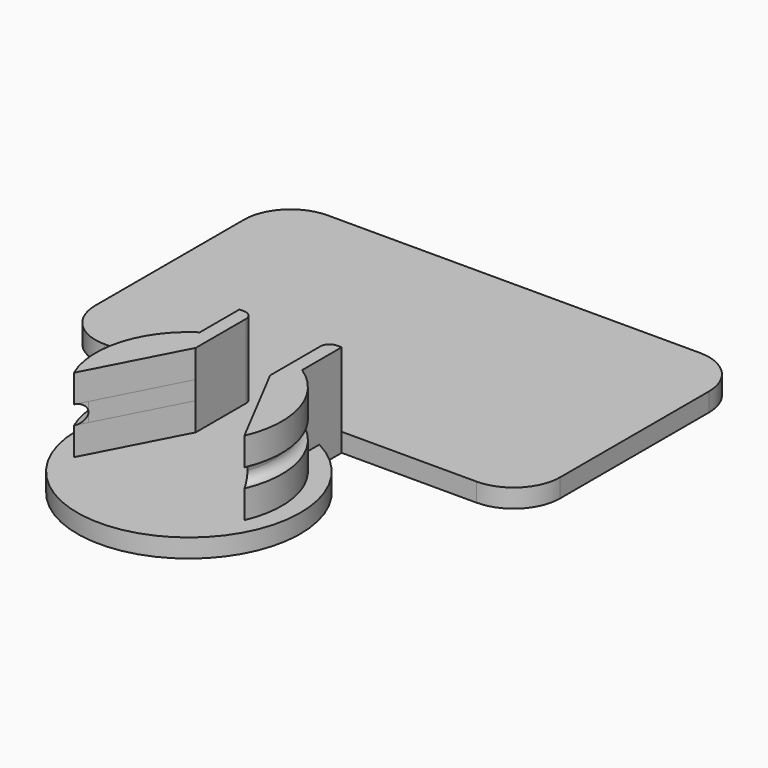
from build123d import *

# Parameters (mm, degrees)
F1_DEPTH     = 2
F3_DEPTH     = 3
F5_DEPTH     = 2
F7_DEPTH     = 3
F8_T4_ANGLE  = 102.3969146675
F8_T10_ANGLE = 102.3969146675
F8_T16_ANGLE = 102.3969146675
F8_T22_ANGLE = 102.3969146675
F8_T26_ANGLE = 121.7069479791
F8_T28_ANGLE = 121.7069479791
F8_T30_ANGLE = 121.7069479791
F8_T32_ANGLE = 121.7069479791
F9_W         = 24
F9_H         = 22.6653645039
F10_DEPTH    = 8
F11_W        = 50
F11_H        = 30
F12_DEPTH    = 2
F13_R        = 1
F14_R        = 5


# Not quite as in the source:
# - a fillet or chamfer that OpenCascade refuses, or shapes differently, is made with other operations: its cross-section is extruded or revolved along the edge and cut away or added


with BuildPart() as f1:
    # F0 (on Top) → F1 (new body)
    with BuildSketch(Plane.XY):
        with BuildLine():
            ThreePointArc((5.5, 1.5), (0, 24.1653645039), (-5.5, 1.5))
            Line((-5.5, 1.5), (-5.5, -1.5))
            ThreePointArc((-5.5, -1.5), (0, -24.1653645039), (5.5, -1.5))
            Line((5.5, -1.5), (5.5, 1.5))
        make_face()
    extrude(amount=F1_DEPTH)

    # F2 (on face) → F3 (join)
    with BuildSketch(Plane.XY.offset(2)):
        with BuildLine():
            Line((9.7844830762, 19.1125863177), (8.6602540378, 17.1653645039))
            ThreePointArc((8.6602540378, 17.1653645039), (9.4991255677, 9.0402063559), (4, 3.0002131139))
            Line((4, 3.0002131139), (4, -6.2432010007))
            Line((4, -6.2432010007), (9.1651513899, -16.1653645039))
            ThreePointArc((9.1651513899, -16.1653645039), (9.5868378212, -9.3206253964), (5.5, -3.8137179596))
            Line((5.5, -3.8137179596), (5.5, 1.5))
            ThreePointArc((5.5, 1.5), (11.6599594736, 9.3289327537), (9.7844830762, 19.1125863177))
        make_face()
        with BuildLine():
            ThreePointArc((-4, 3.0002131139), (-9.4991255677, 9.0402063559), (-8.6602540378, 17.1653645039))
            Line((-8.6602540378, 17.1653645039), (-9.7844830762, 19.1125863177))
            ThreePointArc((-9.7844830762, 19.1125863177), (-11.6599594736, 9.3289327537), (-5.5, 1.5))
            Line((-5.5, 1.5), (-5.5, -3.8137179596))
            ThreePointArc((-5.5, -3.8137179596), (-9.5868378212, -9.3206253964), (-9.1651513899, -16.1653645039))
            Line((-9.1651513899, -16.1653645039), (-4, -6.2432010007))
            Line((-4, -6.2432010007), (-4, 3.0002131139))
        make_face()
    extrude(amount=F3_DEPTH)

    # F4 (on face) → F5 (join)
    with BuildSketch(Plane.XY.offset(5)):
        with BuildLine():
            Line((-8.0717844057, 16.1461052023), (-9.7844830762, 19.1125863177))
            ThreePointArc((-9.7844830762, 19.1125863177), (-11.6599594736, 9.3289327537), (-5.5, 1.5))
            Line((-5.5, 1.5), (-5.5, -5.0414610795))
            ThreePointArc((-5.5, -5.0414610795), (-8.6043935433, -9.5263473097), (-8.5483759414, -14.980549891))
            Line((-8.5483759414, -14.980549891), (-4, -6.2432010007))
            Line((-4, -6.2432010007), (-4, 4.1031067556))
            ThreePointArc((-4, 4.1031067556), (-8.5258693153, 9.2827350759), (-8.0717844057, 16.1461052023))
        make_face()
        with BuildLine():
            ThreePointArc((5.5, 1.5), (11.6599594736, 9.3289327537), (9.7844830762, 19.1125863177))
            Line((9.7844830762, 19.1125863177), (8.0717844057, 16.1461052023))
            ThreePointArc((8.0717844057, 16.1461052023), (8.5258693153, 9.2827350759), (4, 4.1031067556))
            Line((4, 4.1031067556), (4, -6.2432010007))
            Line((4, -6.2432010007), (8.5483759414, -14.980549891))
            ThreePointArc((8.5483759414, -14.980549891), (8.6043935433, -9.5263473097), (5.5, -5.0414610795))
            Line((5.5, -5.0414610795), (5.5, 1.5))
        make_face()
    extrude(amount=F5_DEPTH)

    # F6 (on face) → F7 (join)
    with BuildSketch(Plane.XY.offset(7)):
        with BuildLine():
            Line((9.7844830762, 19.1125863177), (8.6602540378, 17.1653645039))
            ThreePointArc((8.6602540378, 17.1653645039), (9.4991255677, 9.0402063559), (4, 3.0002131139))
            Line((4, 3.0002131139), (4, -6.2432010007))
            Line((4, -6.2432010007), (9.1651513899, -16.1653645039))
            ThreePointArc((9.1651513899, -16.1653645039), (9.5868378212, -9.3206253964), (5.5, -3.8137179596))
            Line((5.5, -3.8137179596), (5.5, 1.5))
            ThreePointArc((5.5, 1.5), (11.6599594736, 9.3289327537), (9.7844830762, 19.1125863177))
        make_face()
        with BuildLine():
            ThreePointArc((-4, 3.0002131139), (-9.4991255677, 9.0402063559), (-8.6602540378, 17.1653645039))
            Line((-8.6602540378, 17.1653645039), (-9.7844830762, 19.1125863177))
            ThreePointArc((-9.7844830762, 19.1125863177), (-11.6599594736, 9.3289327537), (-5.5, 1.5))
            Line((-5.5, 1.5), (-5.5, -3.8137179596))
            ThreePointArc((-5.5, -3.8137179596), (-9.5868378212, -9.3206253964), (-9.1651513899, -16.1653645039))
            Line((-9.1651513899, -16.1653645039), (-4, -6.2432010007))
            Line((-4, -6.2432010007), (-4, 3.0002131139))
        make_face()
    extrude(amount=F7_DEPTH)

    # F8: fillet of radius 1 on 8 edges, made by hand


with BuildPart() as f8_tool2:
    # F8_s3 → F8_t4 (revolve)
    with BuildSketch(Plane(origin=(-4.1871135562, -1.6705281924, 0), x_dir=(0, 0, 1), z_dir=(0.9288065548, 0.3705649522, 0))):
        with BuildLine():
            ThreePointArc((6, 2.2992702923), (5.2928932188, 2.0063770734), (5, 1.2992702923))
            Line((5, 1.2992702923), (5, 2.2992702923))
            Line((5, 2.2992702923), (6, 2.2992702923))
        make_face()
    revolve(axis=Axis((0, -12.1653645039, 5), (0, 0, 1)), revolution_arc=F8_T4_ANGLE)

    split(bisect_by=Plane(origin=(-0.5900874414, 0.3071800789, 0), x_dir=(0, 0, 1), z_dir=(-0.8870108332, 0.4617486132, 0)), keep=Keep.TOP)

    split(bisect_by=Plane.YZ.offset(-4), keep=Keep.BOTTOM)


with BuildPart() as f1_1:
    add(f1.part)

    # F8_t1: union F8_tool2
    add(f8_tool2.part)


with BuildPart() as f8_tool8:
    # F8_s9 → F8_t10 (revolve)
    with BuildSketch(Plane(origin=(-4.1871135562, -1.6705281924, 0), x_dir=(0, 0, 1), z_dir=(0.9288065548, 0.3705649522, 0))):
        with BuildLine():
            ThreePointArc((7, 1.2992702923), (6.7071067812, 2.0063770734), (6, 2.2992702923))
            Line((6, 2.2992702923), (7, 2.2992702923))
            Line((7, 2.2992702923), (7, 1.2992702923))
        make_face()
    revolve(axis=Axis((0, -12.1653645039, 7), (0, 0, 1)), revolution_arc=F8_T10_ANGLE)

    split(bisect_by=Plane(origin=(-0.5900874414, 0.3071800789, 0), x_dir=(0, 0, 1), z_dir=(-0.8870108332, 0.4617486132, 0)), keep=Keep.TOP)

    split(bisect_by=Plane.YZ.offset(-4), keep=Keep.BOTTOM)


with BuildPart() as f1_2:
    add(f1_1.part)

    # F8_t7: union F8_tool8
    add(f8_tool8.part)


with BuildPart() as f8_tool14:
    # F8_s15 → F8_t16 (revolve)
    with BuildSketch(Plane(origin=(-5.6514123525, -8.3322514997, 0), x_dir=(0, 0, 1), z_dir=(-0.561323531, -0.8275964557, 0))):
        with BuildLine():
            ThreePointArc((6, -15.828705359), (6.7071067812, -16.1215985778), (7, -16.828705359))
            Line((7, -16.828705359), (7, -15.828705359))
            Line((7, -15.828705359), (6, -15.828705359))
        make_face()
    revolve(axis=Axis((0, -12.1653645039, 7), (0, 0, 1)), revolution_arc=F8_T16_ANGLE)

    split(bisect_by=Plane.YZ.offset(4), keep=Keep.TOP)

    split(bisect_by=Plane(origin=(0.5900874414, 0.3071800789, 0), x_dir=(0, 0, 1), z_dir=(0.8870108332, 0.4617486132, 0)), keep=Keep.TOP)


with BuildPart() as f1_3:
    add(f1_2.part)

    # F8_t13: union F8_tool14
    add(f8_tool14.part)


with BuildPart() as f8_tool20:
    # F8_s21 → F8_t22 (revolve)
    with BuildSketch(Plane(origin=(-5.6514123525, -8.3322514997, 0), x_dir=(0, 0, 1), z_dir=(-0.561323531, -0.8275964557, 0))):
        with BuildLine():
            ThreePointArc((5, -16.828705359), (5.2928932188, -16.1215985778), (6, -15.828705359))
            Line((6, -15.828705359), (5, -15.828705359))
            Line((5, -15.828705359), (5, -16.828705359))
        make_face()
    revolve(axis=Axis((0, -12.1653645039, 5), (0, 0, 1)), revolution_arc=F8_T22_ANGLE)

    split(bisect_by=Plane.YZ.offset(4), keep=Keep.TOP)

    split(bisect_by=Plane(origin=(0.5900874414, 0.3071800789, 0), x_dir=(0, 0, 1), z_dir=(0.8870108332, 0.4617486132, 0)), keep=Keep.TOP)


with BuildPart() as f1_4:
    add(f1_3.part)

    # F8_t19: union F8_tool20
    add(f8_tool20.part)

    # F8_s25 → F8_t26 (revolve, cut)
    with BuildSketch(Plane(origin=(-6.0530874143, 6.6819786169, 0), x_dir=(0, 0, 1), z_dir=(-0.6713698624, 0.7411224648, 0))):
        with BuildLine():
            ThreePointArc((7, 18.1674590926), (6.7071067812, 17.4603523114), (6, 17.1674590926))
            Line((6, 17.1674590926), (7, 17.1674590926))
            Line((7, 17.1674590926), (7, 18.1674590926))
        make_face()
    revolve(axis=Axis((0, 12.1653645039, 7), (0, 0, -1)), revolution_arc=F8_T26_ANGLE, mode=Mode.SUBTRACT)

    # F8_s27 → F8_t28 (revolve, cut)
    with BuildSketch(Plane(origin=(-2.1730837017, 0.4014208952, 0), x_dir=(0, 0, 1), z_dir=(0.9833630917, -0.1816508459, 0))):
        with BuildLine():
            ThreePointArc((6, -2.9629704506), (6.7071067812, -2.6700772318), (7, -1.9629704506))
            Line((7, -1.9629704506), (7, -2.9629704506))
            Line((7, -2.9629704506), (6, -2.9629704506))
        make_face()
    revolve(axis=Axis((0, 12.1653645039, 7), (0, 0, -1)), revolution_arc=F8_T28_ANGLE, mode=Mode.SUBTRACT)

    # F8_s29 → F8_t30 (revolve, cut)
    with BuildSketch(Plane(origin=(-2.1730837017, 0.4014208952, 0), x_dir=(0, 0, 1), z_dir=(0.9833630917, -0.1816508459, 0))):
        with BuildLine():
            ThreePointArc((5, -1.9629704506), (5.2928932188, -2.6700772318), (6, -2.9629704506))
            Line((6, -2.9629704506), (5, -2.9629704506))
            Line((5, -2.9629704506), (5, -1.9629704506))
        make_face()
    revolve(axis=Axis((0, 12.1653645039, 5), (0, 0, -1)), revolution_arc=F8_T30_ANGLE, mode=Mode.SUBTRACT)

    # F8_s31 → F8_t32 (revolve, cut)
    with BuildSketch(Plane(origin=(-6.0530874143, 6.6819786169, 0), x_dir=(0, 0, 1), z_dir=(-0.6713698624, 0.7411224648, 0))):
        with BuildLine():
            ThreePointArc((6, 17.1674590926), (5.2928932188, 17.4603523114), (5, 18.1674590926))
            Line((5, 18.1674590926), (5, 17.1674590926))
            Line((5, 17.1674590926), (6, 17.1674590926))
        make_face()
    revolve(axis=Axis((0, 12.1653645039, 5), (0, 0, -1)), revolution_arc=F8_T32_ANGLE, mode=Mode.SUBTRACT)

    # F9 (on face) → F10 (cut)
    with BuildSketch(Plane.XY.offset(10)):
        with Locations((0, 12.8326822519)):
            Rectangle(F9_W, F9_H)
    extrude(amount=-F10_DEPTH, mode=Mode.SUBTRACT)

    # F11 (on face) → F12 (join)
    with BuildSketch(Plane.XY.offset(2)):
        with Locations((0, 16.5)):
            Rectangle(F11_W, F11_H)
    extrude(amount=-F12_DEPTH)

    # F13
    f13_edges = [f1_4.edges().sort_by_distance(p)[0] for p in [
        (-4, 1.5, 6),
        (4, 1.5, 6),
    ]]
    fillet(f13_edges, radius=F13_R)

    # F14
    f14_edges = [f1_4.edges().sort_by_distance(p)[0] for p in [
        (-25, 1.5, 1),
        (-25, 31.5, 1),
        (25, 31.5, 1),
        (25, 1.5, 1),
    ]]
    fillet(f14_edges, radius=F14_R)


solid = f1_4.part
